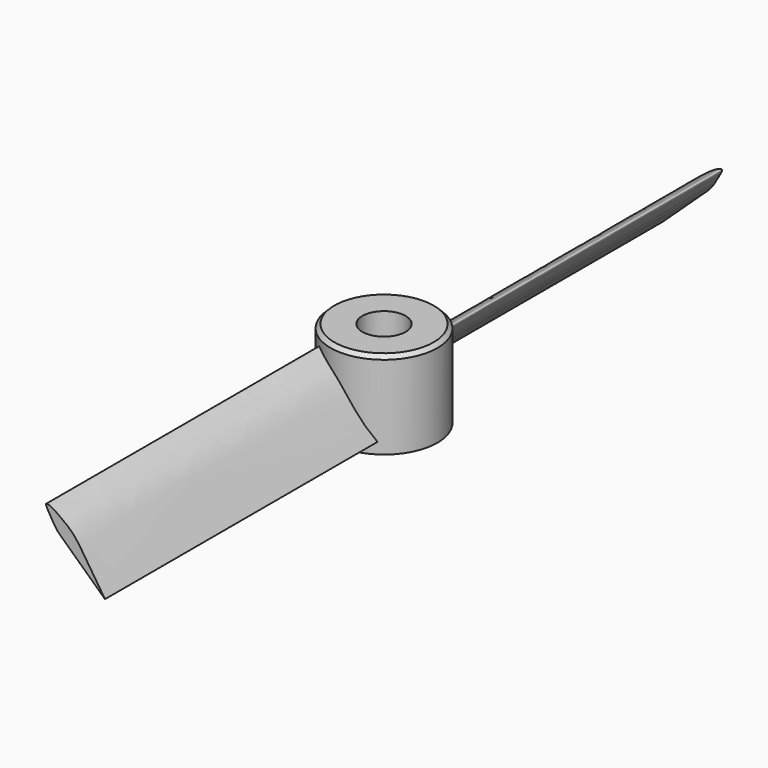
from build123d import *

# Parameters (mm, degrees)
F0_R     = 7.05
F0_R_2   = 2.85
F1_DEPTH = 11.5
F3_DEPTH = 50.8
F4_R     = 5
F6_DEPTH = 50.8
F7_R     = 5
F8_DEPTH = 25
F9_SIZE  = 0.5


# Not quite as in the source:
# - a feature names something its author has since deleted; it is built from what else it names


with BuildPart() as f1:
    # F0 (on Top) → F1 (new body)
    with BuildSketch(Plane.XY):
        Circle(F0_R)
        Circle(F0_R_2, mode=Mode.SUBTRACT)
        Circle(F0_R_2)
    extrude(amount=F1_DEPTH)

    # F2 (on Front) → F3 (join)
    with BuildSketch(Plane.XZ):
        with BuildLine():
            add(Edge.make_bspline(
                [(-2.5891504858, 7.4832015837), (-3.2666322949, 8.7651533189), (-4.9286231356, 11.0050647407), (-1.0780342653, 8.5741441522), (0.3960474288, 6.8659200901), (2.1374814031, 4.0609571357), (3.2837031791, 2.3268894658), (3.8618664427, 1.461158277)],
                knots=[0, 0, 0, 0, 0.1977876363, 0.3919769243, 0.5835513721, 0.7917756861, 1, 1, 1, 1], degree=3))
            Line((-2.5891504858, 7.4832015837), (3.8618664427, 1.461158277))
        make_face()
    extrude(amount=F3_DEPTH)

    # F4
    f4_edges = [f1.edges().sort_by_distance(p)[0] for p in [
        (-2.58915, -28.678674, 7.483202),
    ]]
    fillet(f4_edges, radius=F4_R)

    # F5 (on Front) → F6 (join)
    with BuildSketch(Plane.XZ):
        with BuildLine():
            Line((-3.8620166111, 1.4607873149), (2.5890003174, 7.4828306216))
            add(Edge.make_bspline(
                [(2.5890003174, 7.4828306216), (3.2664821265, 8.7647823568), (4.9284729672, 11.0046937785), (1.077884097, 8.5737731901), (-0.3961975972, 6.865549128), (-2.1376315715, 4.0605861736), (-3.2838533475, 2.3265185037), (-3.8620166111, 1.4607873149)],
                knots=[0, 0, 0, 0, 0.1977876363, 0.3919769243, 0.5835513721, 0.7917756861, 1, 1, 1, 1], degree=3))
        make_face()
    extrude(amount=-F6_DEPTH)

    # F7
    f7_edges = [f1.edges().sort_by_distance(p)[0] for p in [
        (2.589, 28.678703, 7.482831),
    ]]
    fillet(f7_edges, radius=F7_R)

    # F0 (on Top) → F8 (cut)
    with BuildSketch(Plane.XY):
        Circle(F0_R_2)
    extrude(amount=F8_DEPTH, mode=Mode.SUBTRACT)

    # F9
    f9_edges = [f1.edges().sort_by_distance(p)[0] for p in [
        (-7.05, 0, 11.5),
    ]]
    chamfer(f9_edges, length=F9_SIZE)


solid = f1.part
